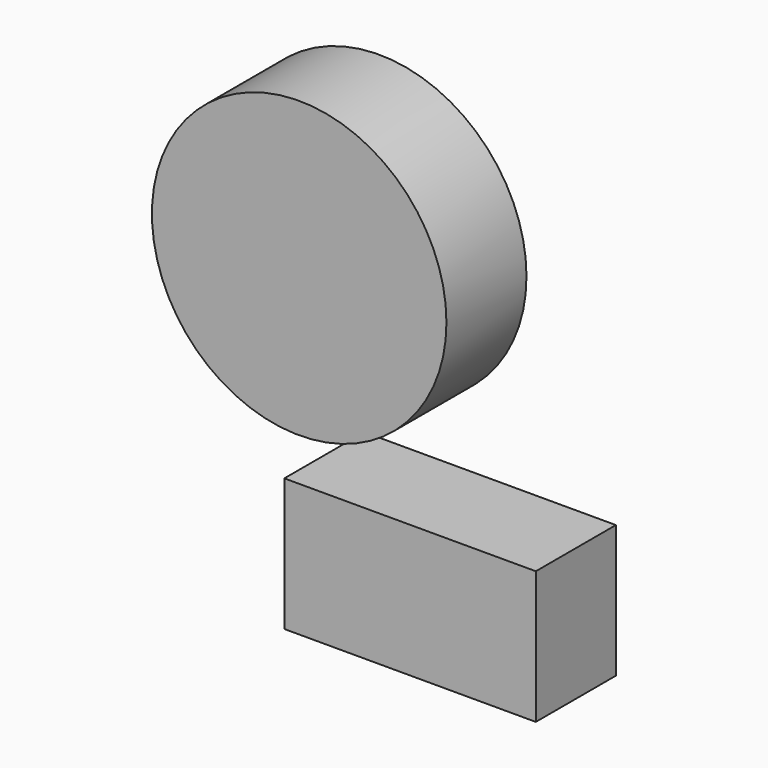
from build123d import *

# Parameters (mm, degrees)
F0_R     = 37.3846562125
F1_DEPTH = 25.4
F0_W     = 63.8463646173
F0_H     = 33.6742438376
F3_DEPTH = 3683
F4_R     = 7.4510701555
F5_DEPTH = 3683


# Not quite as in the source:
# - a feature names something its author has since deleted; it is built from what else it names


with BuildPart() as f1:
    # F0 (on Front) → F1 (new body)
    with BuildSketch(Plane.XZ):
        with Locations((-19.9351515621, 24.7842408717)):
            Circle(F0_R)
    extrude(amount=F1_DEPTH)

    # F0 (on Front) → F3 (cut)
    with BuildSketch(Plane.XZ):
        with Locations((-19.9351515621, 24.7842408717)):
            Circle(F0_R)
        with Locations((8.2165151834, -40.2743946761)):
            Rectangle(F0_W, F0_H)
    extrude(amount=-F3_DEPTH, mode=Mode.SUBTRACT)

    # F4 (on Front) + F0 (on Front) → F5 (cut)
    with BuildSketch(Plane.XZ):
        with Locations((-10.7757588848, 47.1439398825)):
            Circle(F4_R)
    with BuildSketch(Plane.XZ):
        with Locations((-19.9351515621, 24.7842408717)):
            Circle(F0_R)
        with Locations((8.2165151834, -40.2743946761)):
            Rectangle(F0_W, F0_H)
    extrude(amount=-F5_DEPTH, mode=Mode.SUBTRACT)


with BuildPart() as f1b:
    # F0 (on Front) → F1, piece 2 (new body)
    with BuildSketch(Plane.XZ):
        with Locations((8.2165151834, -40.2743946761)):
            Rectangle(F0_W, F0_H)
    extrude(amount=F1_DEPTH)


solid = Compound([f1.part, f1b.part])
